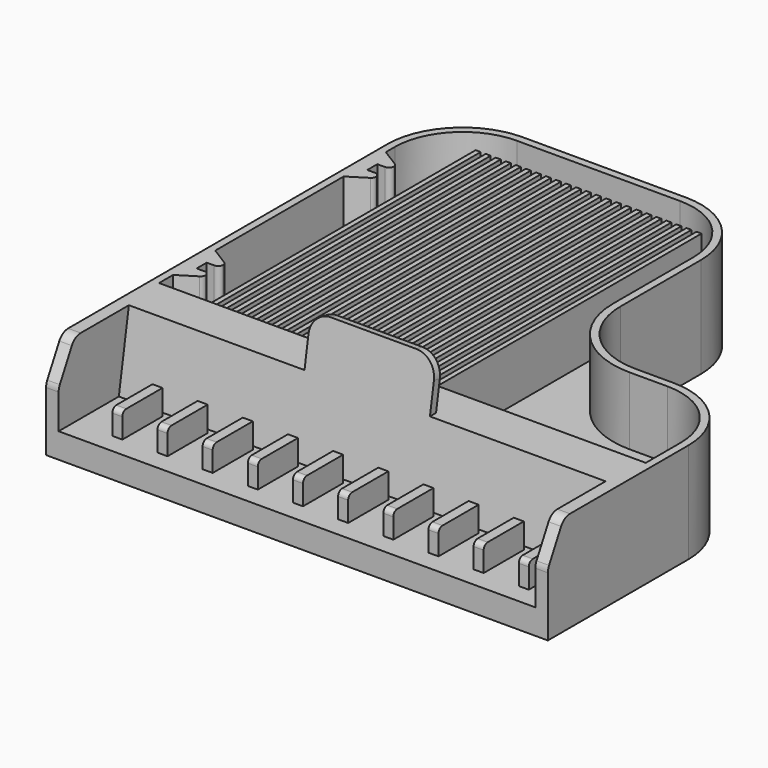
from build123d import *

# Parameters (mm, degrees)
F1_DEPTH     = 40
F4_START     = 8
F4_DEPTH     = 27.7
F6_DEPTH     = 95
F7_W         = 20
F7_H         = 12
F8_DEPTH     = 5
F9_SIZE2     = 15
F9_SIZE      = 8
F10_R        = 5
F11_W        = 4
F11_H        = 20
F12_DEPTH    = 10
F13_R        = 2
F14_W        = 20
F14_H        = 20
F14_W_2      = 30
F15_DEPTH    = 3
F16_R        = 8
F18_DEPTH    = 27
F19_T1_DEPTH = 29.7712382075
F19_T3_DEPTH = 32
F20_W        = 2
F20_H        = 135
F21_DEPTH    = 22


# Not quite as in the source:
# - a fillet or chamfer that OpenCascade refuses, or shapes differently, is made with other operations: its cross-section is extruded or revolved along the edge and cut away or added


with BuildPart() as f1:
    # F0 (on Top) → F1 (new body)
    with BuildSketch(Plane.XY):
        with BuildLine():
            ThreePointArc((70, 100), (48.7867965644, 48.7867965644), (100, 70))
            ThreePointArc((100, 70), (91.2132034356, 91.2132034356), (70, 100))
        make_face()
        with BuildLine():
            ThreePointArc((-70, 200), (-91.2132034356, 191.2132034356), (-100, 170))
            ThreePointArc((-100, 170), (-70, 140), (-40, 170))
            ThreePointArc((-40, 170), (-48.7867965644, 191.2132034356), (-70, 200))
        make_face()
        with BuildLine():
            ThreePointArc((25, 170), (16.2132035072, 191.213203364), (-4.9999997975, 200))
            ThreePointArc((-4.9999997975, 200), (-26.2132035072, 148.786796636), (25, 170))
        make_face()
        with BuildLine():
            Line((-100, 170), (-100, 0))
            Line((-100, 0), (100, 0))
            Line((100, 0), (100, 70))
            ThreePointArc((100, 70), (48.7867965644, 48.7867965644), (70, 100))
            Line((70, 100), (55, 100))
            Line((55, 100), (25, 100))
            Line((25, 100), (25, 130))
            Line((25, 130), (25, 170))
            ThreePointArc((25, 170), (-26.2132035072, 148.786796636), (-4.9999997975, 200))
            Line((-4.9999997975, 200), (-70, 200))
            ThreePointArc((-70, 200), (-48.7867965644, 191.2132034356), (-40, 170))
            ThreePointArc((-40, 170), (-70, 140), (-100, 170))
        make_face()
        with BuildLine():
            Line((25, 100), (55, 100))
            ThreePointArc((55, 100), (33.7867965644, 108.7867965644), (25, 130))
            Line((25, 130), (25, 100))
        make_face()
    extrude(amount=F1_DEPTH)

    # F3 (on offset) → F4 (cut)
    with BuildSketch(Plane.XY.offset(5).offset(F4_START)):
        with BuildLine():
            Line((-5, 197), (-70, 197))
            ThreePointArc((-70, 197), (-89.091883092, 189.091883092), (-97, 170))
            Line((-97, 170), (-97, 52.5304101706))
            Line((-97, 52.5304101706), (97, 52.5304101706))
            Line((97, 52.5304101706), (97, 70))
            ThreePointArc((97, 70), (89.091883092, 89.091883092), (70, 97))
            Line((70, 97), (55, 97))
            ThreePointArc((55, 97), (31.6654762208, 106.6654762208), (22, 130))
            Line((22, 130), (22, 170))
            ThreePointArc((22, 170), (14.091883092, 189.091883092), (-5, 197))
        make_face()
    extrude(amount=F4_DEPTH, mode=Mode.SUBTRACT)

    # F5 (on Right) → F6 (cut, symmetric)
    with BuildSketch(Plane.YZ):
        Polygon((35, 40), (0, 40), (0, 10), (30, 10), align=None)
    extrude(amount=F6_DEPTH, both=True, mode=Mode.SUBTRACT)

    # F7 (on face) → F8 (cut)
    with BuildSketch(Plane(origin=(0, 0, 0), x_dir=(1, 0, 0), z_dir=(0, 0, -1))):
        with Locations((80, -30)):
            Rectangle(F7_W, F7_H)
        with Locations((-80, -30)):
            Rectangle(F7_W, F7_H)
        with Locations((-37.5, -170)):
            Rectangle(F7_W, F7_H)
    extrude(amount=-F8_DEPTH, mode=Mode.SUBTRACT)

    # F9
    f9_edges = [f1.edges().sort_by_distance(p)[0] for p in [
        (-97.5, 0, 40),
        (97.5, 0, 40),
    ]]
    chamfer(f9_edges, length=F9_SIZE, length2=F9_SIZE2)

    # F10
    f10_edges = [f1.edges().sort_by_distance(p)[0] for p in [
        (97.5, 8, 40),
        (97.5, 0, 25),
        (-97.5, 0, 25),
        (-97.5, 8, 40),
    ]]
    fillet(f10_edges, radius=F10_R)

    # F11 (on face) → F12 (join)
    with BuildSketch(Plane.XY.offset(10)):
        with Locations((-78, 18)):
            Rectangle(F11_W, F11_H)
        with Locations((-60, 18)):
            Rectangle(F11_W, F11_H)
        with Locations((-42, 18)):
            Rectangle(F11_W, F11_H)
        with Locations((-24, 18)):
            Rectangle(F11_W, F11_H)
        with Locations((-6, 18)):
            Rectangle(F11_W, F11_H)
        with Locations((12, 18)):
            Rectangle(F11_W, F11_H)
        with Locations((30, 18)):
            Rectangle(F11_W, F11_H)
        with Locations((48, 18)):
            Rectangle(F11_W, F11_H)
        with Locations((66, 18)):
            Rectangle(F11_W, F11_H)
        with Locations((84, 18)):
            Rectangle(F11_W, F11_H)
    extrude(amount=F12_DEPTH)

    # F13
    f13_edges = [f1.edges().sort_by_distance(p)[0] for p in [
        (-78, 8, 20),
        (-60, 8, 20),
        (-42, 8, 20),
        (-24, 8, 20),
        (-6, 8, 20),
        (12, 8, 20),
        (30, 8, 20),
        (48, 8, 20),
        (66, 8, 20),
        (84, 8, 20),
    ]]
    fillet(f13_edges, radius=F13_R)

    # F14 (on face) → F15 (join)
    with BuildSketch(Plane(origin=(0, 27.5675675676, -4.5945945946), x_dir=(1, 0, 0), z_dir=(0, -0.9863939238, 0.1643989873))):
        with Locations((-15, 55.209721509)):
            Rectangle(F14_W, F14_H)
        with Locations((10, 55.209721509)):
            Rectangle(F14_W_2, F14_H)
    extrude(amount=-F15_DEPTH)

    # F16
    f16_edges = [f1.edges().sort_by_distance(p)[0] for p in [
        (-25, 39.767571, 59.48128),
        (25, 39.767571, 59.48128),
    ]]
    fillet(f16_edges, radius=F16_R)

    # F17 (on face) → F18 (join)
    with BuildSketch(Plane.XY.offset(13)):
        Polygon((-89, 160.5304101706), (-97, 165.5304101706), (-97, 144.5304101706), (-89, 149.5304101706), (-89, 152.5304101706), (-94, 152.5304101706), (-94, 157.5304101706), (-89, 157.5304101706), align=None)
        Polygon((-89, 64.5304101706), (-89, 67.5304101706), (-94, 67.5304101706), (-94, 72.5304101706), (-89, 72.5304101706), (-89, 75.5304101706), (-97, 80.5304101706), (-97, 59.5304101706), align=None)
    extrude(amount=F18_DEPTH)

    # F19: fillet of radius 2 on 8 edges, made by hand

    # F19_s2 → F19_t1 (cut)
    with BuildSketch(Plane.XY.offset(13)):
        with BuildLine():
            ThreePointArc((-89.94000212, 63.9429088456), (-89.2507150375, 64.6693683888), (-89, 65.6389054536))
            Line((-89, 65.6389054536), (-89, 64.5304101706))
            Line((-89, 64.5304101706), (-89.94000212, 63.9429088456))
        make_face()
        with BuildLine():
            ThreePointArc((-89, 74.4219148875), (-89.2507150375, 75.3914519523), (-89.94000212, 76.1179114956))
            Line((-89.94000212, 76.1179114956), (-89, 75.5304101706))
            Line((-89, 75.5304101706), (-89, 74.4219148875))
        make_face()
        with BuildLine():
            ThreePointArc((-89.94000212, 148.9429088456), (-89.2507150375, 149.6693683888), (-89, 150.6389054536))
            Line((-89, 150.6389054536), (-89, 149.5304101706))
            Line((-89, 149.5304101706), (-89.94000212, 148.9429088456))
        make_face()
        with BuildLine():
            ThreePointArc((-89.94000212, 161.1179114956), (-89.2507150375, 160.3914519523), (-89, 159.4219148875))
            Line((-89, 159.4219148875), (-89, 160.5304101706))
            Line((-89, 160.5304101706), (-89.94000212, 161.1179114956))
        make_face()
    extrude(amount=F19_T1_DEPTH, mode=Mode.SUBTRACT)

    # F19_s4 → F19_t3 (cut)
    with BuildSketch(Plane.XY.offset(13)):
        with BuildLine():
            ThreePointArc((-91, 72.5304101706), (-89.5857864376, 73.1161966082), (-89, 74.5304101706))
            Line((-89, 74.5304101706), (-89, 72.5304101706))
            Line((-89, 72.5304101706), (-91, 72.5304101706))
        make_face()
        with BuildLine():
            ThreePointArc((-89, 65.5304101706), (-89.5857864376, 66.9446237329), (-91, 67.5304101706))
            Line((-91, 67.5304101706), (-89, 67.5304101706))
            Line((-89, 67.5304101706), (-89, 65.5304101706))
        make_face()
        with BuildLine():
            ThreePointArc((-89, 150.5304101706), (-89.5857864376, 151.9446237329), (-91, 152.5304101706))
            Line((-91, 152.5304101706), (-89, 152.5304101706))
            Line((-89, 152.5304101706), (-89, 150.5304101706))
        make_face()
        with BuildLine():
            ThreePointArc((-91, 157.5304101706), (-89.5857864376, 158.1161966082), (-89, 159.5304101706))
            Line((-89, 159.5304101706), (-89, 157.5304101706))
            Line((-89, 157.5304101706), (-91, 157.5304101706))
        make_face()
    extrude(amount=F19_T3_DEPTH, mode=Mode.SUBTRACT)

    # F20 (on face) → F21 (join)
    with BuildSketch(Plane.XY.offset(13)):
        with Locations((-81.000735837, 124.0304101706)):
            Rectangle(F20_W, F20_H)
        with Locations((-77.000735837, 124.0304101706)):
            Rectangle(F20_W, F20_H)
        with Locations((-73.000735837, 124.0304101706)):
            Rectangle(F20_W, F20_H)
        with Locations((-69.000735837, 124.0304101706)):
            Rectangle(F20_W, F20_H)
        with Locations((-65.000735837, 124.0304101706)):
            Rectangle(F20_W, F20_H)
        with Locations((-61.000735837, 124.0304101706)):
            Rectangle(F20_W, F20_H)
        with Locations((-57.000735837, 124.0304101706)):
            Rectangle(F20_W, F20_H)
        with Locations((-53.000735837, 124.0304101706)):
            Rectangle(F20_W, F20_H)
        with Locations((-49.000735837, 124.0304101706)):
            Rectangle(F20_W, F20_H)
        with Locations((-45.000735837, 124.0304101706)):
            Rectangle(F20_W, F20_H)
        with Locations((-41.000735837, 124.0304101706)):
            Rectangle(F20_W, F20_H)
        with Locations((-37.000735837, 124.0304101706)):
            Rectangle(F20_W, F20_H)
        with Locations((-33.000735837, 124.0304101706)):
            Rectangle(F20_W, F20_H)
        with Locations((-29.000735837, 124.0304101706)):
            Rectangle(F20_W, F20_H)
        with Locations((-25.000735837, 124.0304101706)):
            Rectangle(F20_W, F20_H)
        with Locations((-21.000735837, 124.0304101706)):
            Rectangle(F20_W, F20_H)
        with Locations((-17.000735837, 124.0304101706)):
            Rectangle(F20_W, F20_H)
        with Locations((-13.000735837, 124.0304101706)):
            Rectangle(F20_W, F20_H)
        with Locations((-9.000735837, 124.0304101706)):
            Rectangle(F20_W, F20_H)
        with Locations((-5.000735837, 124.0304101706)):
            Rectangle(F20_W, F20_H)
        with Locations((-1.000735837, 124.0304101706)):
            Rectangle(F20_W, F20_H)
        with Locations((2.999264163, 124.0304101706)):
            Rectangle(F20_W, F20_H)
        with Locations((6.999264163, 124.0304101706)):
            Rectangle(F20_W, F20_H)
    extrude(amount=F21_DEPTH)


solid = f1.part
